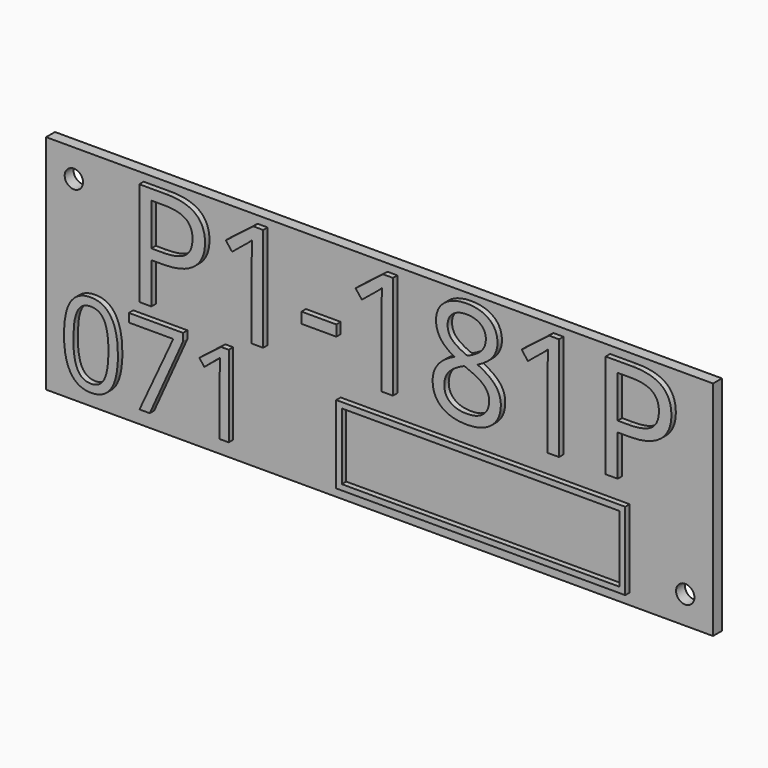
from build123d import *

# Parameters (mm, degrees)
F0_W         = 120
F0_H         = 40
F1_DEPTH     = 2
F3_D         = 3.3
F4_TEXT_SIZE = 26.1352499183
F5_DEPTH     = 1
F6_TEXT_SIZE = 20.5478077656
F7_DEPTH     = 1
F8_W         = 52
F8_H         = 14
F8_W_2       = 49.99999962
F8_H_2       = 11.99999962
F9_DEPTH     = 1


# Not quite as in the source:
# - Text() gives the source's letters only with a copy of the font that has no kerning and outlines rounded to 1/6400 em; it was checked with that copy


with BuildPart() as f1:
    # F0 (on Front) → F1 (new body)
    with BuildSketch(Plane.XZ):
        Rectangle(F0_W, F0_H)
    extrude(amount=F1_DEPTH)

    # F3 (through all)
    with Locations(Plane.XZ.offset(2)):
        with Locations((-55, 15), (55, -15)):
            Hole(F3_D / 2)

    # F4 (on face) → F5 (join)
    with BuildSketch(Plane.XZ.offset(2)):
        with Locations((-45, 0)):
            Text('P1-181P', F4_TEXT_SIZE, font='Open Sans', text_align=(TextAlign.LEFT, TextAlign.BOTTOM))
    extrude(amount=F5_DEPTH)

    # F6 (on face) → F7 (join)
    with BuildSketch(Plane.XZ.offset(2)):
        with Locations((-57, -17)):
            Text('071', F6_TEXT_SIZE, font='Open Sans', text_align=(TextAlign.LEFT, TextAlign.BOTTOM))
    extrude(amount=F7_DEPTH)

    # F8 (on face) → F9 (join)
    with BuildSketch(Plane.XZ.offset(2)):
        with Locations((19, -11)):
            Rectangle(F8_W, F8_H)
        with Locations((19, -11)):
            Rectangle(F8_W_2, F8_H_2, mode=Mode.SUBTRACT)
    extrude(amount=F9_DEPTH)


solid = f1.part
